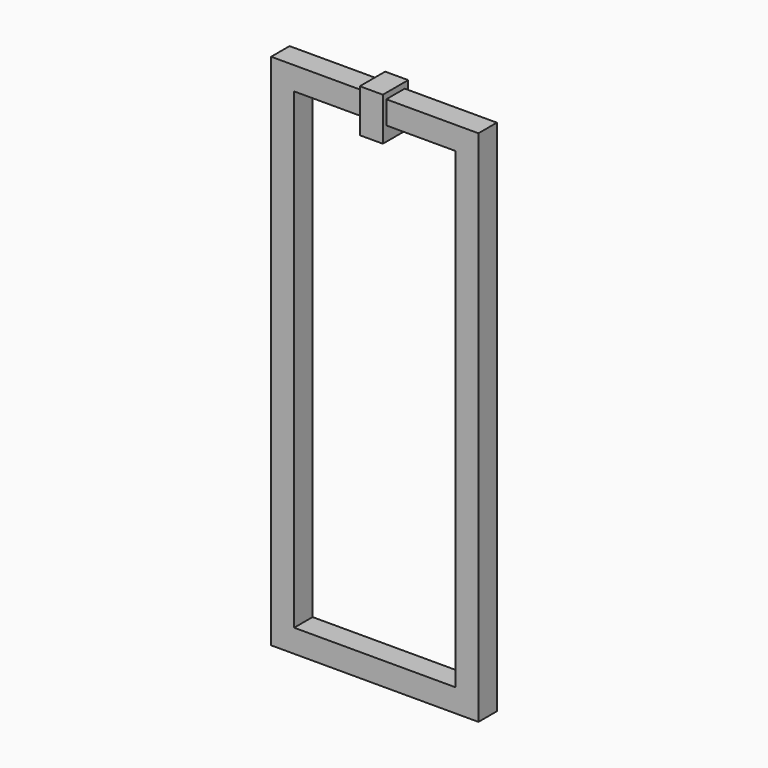
from build123d import *

# Parameters (mm, degrees)
F0_W          = 914.4
F0_H          = 101.6
F1_DEPTH      = 2286
F2_T          = -101.6
F3_W          = 101.6
F3_H          = 139.7
F4_DEPTH      = 165.1
F4_DEPTH_BACK = 25.4
F5_T          = 50.8
F5_T3_DEPTH   = 203.2
F6_SIZE       = 5.08


# Not quite as in the source:
# - a shell that OpenCascade refuses in one call is made with other operations: the cavity is built on its own and cut out


with BuildPart() as f1:
    # F0 (on Top) → F1 (new body)
    with BuildSketch(Plane.XY):
        Rectangle(F0_W, F0_H)
    extrude(amount=F1_DEPTH)

    # F2
    f2_openings = [f1.faces().sort_by_distance(p)[0] for p in [
        (0, -50.8, 1143),
        (0, 50.8, 1143),
    ]]
    offset(amount=F2_T, openings=f2_openings)

    # F3 (on face) → F4 (join, two sides)
    with BuildSketch(Plane.XY.offset(2286)) as f4_sk:
        Rectangle(F3_W, F3_H)
    extrude(amount=-F4_DEPTH)
    extrude(f4_sk.sketch, amount=F4_DEPTH_BACK)

    # F5: shell of thickness 50.8, made by hand


with BuildPart() as f5_core1:
    # F5_t2: copy of F1
    add(f1.part)

    # the walls: a layer under each face that stays
    f5_faces = [f5_core1.faces().sort_by_distance(p)[0] for p in [
        (-457.2, 0, 1143),
        (391.8857142857, 50.8, 2122.7142857143),
        (-391.8857142857, -50.8, 2122.7142857143),
        (0, 0, 0),
        (-254, 0, 2286),
        (-203.2, 0, 2184.4),
        (-355.6, 0, 1143),
        (0, 0, 101.6),
        (355.6, 0, 1143),
        (203.2, 0, 2184.4),
        (254, 0, 2286),
        (457.2, 0, 1143),
        (0, 0, 2120.9),
        (0, 69.85, 2216.15),
        (0, -69.85, 2216.15),
        (0, 0, 2311.4),
    ]]
    thicken(f5_faces, amount=-F5_T, mode=Mode.SUBTRACT)

    # F5_s4 → F5_t3 (cut)
    with BuildSketch(Plane.XZ.offset(-101.6)):
        Polygon((-355.092, 2183.892), (-355.6, 2235.2), (-406.4, 2235.2), (-406.4, 2184.4), align=None)
        Polygon((-355.092, 102.108), (-406.4, 101.6), (-406.4, 50.8), (-355.6, 50.8), align=None)
        Polygon((355.092, 102.108), (355.6, 50.8), (406.4, 50.8), (406.4, 101.6), align=None)
        Polygon((355.092, 2183.892), (406.4, 2184.4), (406.4, 2235.2), (355.6, 2235.2), align=None)
    extrude(amount=F5_T3_DEPTH, mode=Mode.SUBTRACT)


with BuildPart() as f1_1:
    add(f1.part)

    # what is left inside the walls is the cavity
    f5_cavity = [f5_core1.part.solids().sort_by_distance(p)[0] for p in [
        (0, -18.542, 2201.333333),
    ]]
    add(f5_cavity, mode=Mode.SUBTRACT)

    # F6
    f6_edges = [f1_1.edges().sort_by_distance(p)[0] for p in [
        (-50.8, 0, 2171.7),
    ]]
    chamfer(f6_edges, length=F6_SIZE)


solid = f1_1.part
